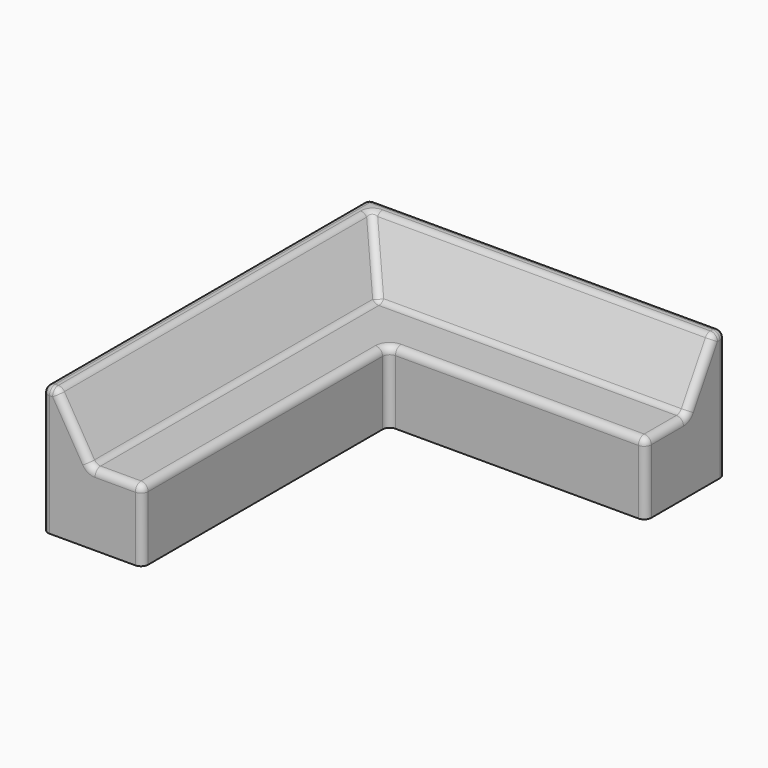
from build123d import *

# Parameters (mm, degrees)
F0_W         = 18
F0_H         = 7
F1_DEPTH     = 5
F2_W         = 21
F2_H         = 4
F3_DEPTH     = 4
F4_T4_DEPTH  = 37.431305486
F4_T9_DEPTH  = 33.931305486
F4_T15_DEPTH = 33.931305486
F4_T21_DEPTH = 37.431305486
F5_R         = 0.5
F6_T1_DEPTH  = 2.8169048105
F6_T3_DEPTH  = 2.8169048105
F6_T5_DEPTH  = 0.2169048105
F6_T7_DEPTH  = 4.0985711369
F6_T9_DEPTH  = 0.2169048105
F6_T11_DEPTH = 4.0985711369
F6_S15_W     = 0.5
F6_S15_H     = 0.5
F6_T16_DEPTH = 0.5
F6_S21_W     = 0.5
F6_S21_H     = 0.5
F6_T22_DEPTH = 0.5
F6_S27_W     = 0.5
F6_S27_H     = 0.5
F6_T28_DEPTH = 0.5
F6_S33_W     = 0.5
F6_S33_H     = 0.5
F6_T34_DEPTH = 0.5
F6_T38_ANGLE = 59.0362434679
F6_T40_ANGLE = 59.0362434679
F6_T42_ANGLE = 59.0362434679
F6_T44_ANGLE = 59.0362434679


# Not quite as in the source:
# - a fillet or chamfer that OpenCascade refuses, or shapes differently, is made with other operations: its cross-section is extruded or revolved along the edge and cut away or added


with BuildPart() as f1:
    # F0 (on Top) → F1 (new body)
    with BuildSketch(Plane.XY):
        Polygon((-41.0881050097, 20.8523701802), (-48.0881050097, 20.8523701802), (-48.0881050097, -7.6476298198), (-41.0881050097, -7.6476298198), (-41.0881050097, 13.8523701802), align=None)
        with Locations((-32.0881050097, 17.3523701802)):
            Rectangle(F0_W, F0_H)
    extrude(amount=F1_DEPTH)

    # F2 (on face) → F3 (join)
    with BuildSketch(Plane.XY.offset(5)):
        Polygon((-44.0881050097, 20.8523701802), (-48.0881050097, 20.8523701802), (-48.0881050097, -7.6476298198), (-44.0881050097, -7.6476298198), (-44.0881050097, 16.8523701802), align=None)
        with Locations((-33.5881050097, 18.8523701802)):
            Rectangle(F2_W, F2_H)
    extrude(amount=F3_DEPTH)

    # F4: chamfer of 5 x 3 on 2 edges, made by hand


with BuildPart() as f4_tool2:
    # F4_s3 → F4_t4 (new body)
    with BuildSketch(Plane.XZ.offset(20.5789353058)):
        Polygon((-44.0881050097, 4), (-47.0881050097, 9), (-44.0881050097, 9), align=None)
    extrude(amount=-F4_T4_DEPTH)

    split(bisect_by=Plane.XY.offset(5), keep=Keep.TOP)


with BuildPart() as f1_1:
    add(f1.part)

    # F4_t1: cut F4_tool2
    add(f4_tool2.part, mode=Mode.SUBTRACT)


with BuildPart() as f4_tool7:
    # F4_s8 → F4_t9 (new body)
    with BuildSketch(Plane.YZ.offset(-44.0881050097)):
        Polygon((16.8523701802, 4), (19.8523701802, 9), (16.8523701802, 9), align=None)
    extrude(amount=F4_T9_DEPTH)

    split(bisect_by=Plane.XY.offset(5), keep=Keep.TOP)


with BuildPart() as f1_2:
    add(f1_1.part)

    # F4_t6: cut F4_tool7
    add(f4_tool7.part, mode=Mode.SUBTRACT)


with BuildPart() as f4_tool13:
    # F4_s14 → F4_t15 (new body)
    with BuildSketch(Plane.YZ.offset(-57.0194104957)):
        Polygon((16.8523701802, 4), (19.8523701802, 9), (16.8523701802, 9), align=None)
    extrude(amount=F4_T15_DEPTH)

    split(bisect_by=Plane.YZ.offset(-48.0881050097), keep=Keep.TOP)

    split(bisect_by=Plane.YZ.offset(-44.0881050097), keep=Keep.BOTTOM)

    split(bisect_by=Plane.XY.offset(5), keep=Keep.TOP)


with BuildPart() as f4_tool19:
    # F4_s20 → F4_t21 (new body)
    with BuildSketch(Plane.XZ.offset(7.6476298198)):
        Polygon((-44.0881050097, 4), (-47.0881050097, 9), (-44.0881050097, 9), align=None)
    extrude(amount=-F4_T21_DEPTH)

    split(bisect_by=Plane.XZ.offset(-16.8523701802), keep=Keep.BOTTOM)

    split(bisect_by=Plane.XY.offset(5), keep=Keep.TOP)

    split(bisect_by=Plane.XZ.offset(-20.8523701802), keep=Keep.TOP)


with BuildPart() as f4_tool13_1:
    add(f4_tool13.part)

    # F4_t25: intersect F4_tool19
    add(f4_tool19.part, mode=Mode.INTERSECT)


with BuildPart() as f1_3:
    add(f1_2.part)

    # F4_t11: cut F4_tool13
    add(f4_tool13_1.part, mode=Mode.SUBTRACT)

    # F5
    f5_edges = [f1_3.edges().sort_by_distance(p)[0] for p in [
        (-48.088105, -7.64763, 4.5),
        (-41.088105, -7.64763, 2.5),
        (-41.088105, 13.85237, 2.5),
        (-23.088105, 13.85237, 2.5),
        (-23.088105, 20.85237, 4.5),
        (-35.588105, 20.85237, 9),
        (-35.088105, 19.85237, 9),
        (-47.088105, 6.10237, 9),
        (-45.888105, 18.65237, 7),
        (-33.888105, 17.45237, 5),
        (-44.688105, 4.90237, 5),
        (-41.088105, 3.10237, 5),
        (-32.088105, 13.85237, 5),
        (-48.088105, 6.60237, 9),
        (-48.088105, 20.85237, 4.5),
    ]]
    fillet(f5_edges, radius=F5_R)

    # F6: fillet of radius 0.5 on 10 edges, made by hand

    # F6_s2 → F6_t1 (cut)
    with BuildSketch(Plane.YZ.offset(-44.4050098202)):
        with BuildLine():
            ThreePointArc((-7.6476298198, 4.5), (-7.5011832104, 4.8535533906), (-7.1476298198, 5))
            Line((-7.1476298198, 5), (-7.6476298198, 5))
            Line((-7.6476298198, 5), (-7.6476298198, 4.5))
        make_face()
    extrude(amount=F6_T1_DEPTH, mode=Mode.SUBTRACT)

    # F6_s4 → F6_t3 (cut)
    with BuildSketch(Plane.XZ.offset(-17.1692749907)):
        with BuildLine():
            ThreePointArc((-23.0881050097, 4.5), (-23.2345516191, 4.8535533906), (-23.5881050097, 5))
            Line((-23.5881050097, 5), (-23.0881050097, 5))
            Line((-23.0881050097, 5), (-23.0881050097, 4.5))
        make_face()
    extrude(amount=F6_T3_DEPTH, mode=Mode.SUBTRACT)

    # F6_s6 → F6_t5 (cut)
    with BuildSketch(Plane.YZ.offset(-47.5881050097)):
        with BuildLine():
            ThreePointArc((-7.6476298198, 8.5), (-7.5011832104, 8.8535533906), (-7.1476298198, 9))
            Line((-7.1476298198, 9), (-7.6476298198, 9))
            Line((-7.6476298198, 9), (-7.6476298198, 8.5))
        make_face()
    extrude(amount=F6_T5_DEPTH, mode=Mode.SUBTRACT)

    # F6_s8 → F6_t7 (cut)
    with BuildSketch(Plane(origin=(-16.2894353468, 0, 27.1490589114), x_dir=(0, 1, 0), z_dir=(0.5144957554, 0, -0.8574929257))):
        with BuildLine():
            ThreePointArc((-7.6476298198, -36.2472551322), (-7.5011832104, -35.8937017416), (-7.1476298198, -35.7472551322))
            Line((-7.1476298198, -35.7472551322), (-7.6476298198, -35.7472551322))
            Line((-7.6476298198, -35.7472551322), (-7.6476298198, -36.2472551322))
        make_face()
    extrude(amount=F6_T7_DEPTH, mode=Mode.SUBTRACT)

    # F6_s10 → F6_t9 (cut)
    with BuildSketch(Plane.XZ.offset(-20.3523701802)):
        with BuildLine():
            ThreePointArc((-23.0881050097, 8.5), (-23.2345516191, 8.8535533906), (-23.5881050097, 9))
            Line((-23.5881050097, 9), (-23.0881050097, 9))
            Line((-23.0881050097, 9), (-23.0881050097, 8.5))
        make_face()
    extrude(amount=F6_T9_DEPTH, mode=Mode.SUBTRACT)

    # F6_s12 → F6_t11 (cut)
    with BuildSketch(Plane(origin=(0, 6.971278674, 11.61879779), x_dir=(1, 0, 0), z_dir=(0, 0.5144957554, 0.8574929257))):
        with BuildLine():
            ThreePointArc((-23.0881050097, 12.8928051893), (-23.2345516191, 12.5392517987), (-23.5881050097, 12.3928051893))
            Line((-23.5881050097, 12.3928051893), (-23.0881050097, 12.3928051893))
            Line((-23.0881050097, 12.3928051893), (-23.0881050097, 12.8928051893))
        make_face()
    extrude(amount=F6_T11_DEPTH, mode=Mode.SUBTRACT)


with BuildPart() as f6_tool14:
    # F6_s15 → F6_t16 (new body)
    with BuildSketch(Plane.YZ.offset(-23.5881050097)):
        with Locations((20.6023701802, 8.75)):
            Rectangle(F6_S15_W, F6_S15_H)
    extrude(amount=F6_T16_DEPTH)

    # F6_s17 → F6_t18 (revolve, cut)
    with BuildSketch(Plane(origin=(-23.5881050097, 20.3523701802, 8.5), x_dir=(0, -0.7071067812, -0.7071067812), z_dir=(0, -0.7071067812, 0.7071067812))):
        with BuildLine():
            ThreePointArc((0, -0.5), (0.5, 0), (0, 0.5))
            Line((0, 0.5), (0, -0.5))
        make_face()
    revolve(axis=Axis((-23.5881050097, 20.3523701802, 8.5), (1, 0, 0)), mode=Mode.SUBTRACT)


with BuildPart() as f1_4:
    add(f1_3.part)

    # F6_t13: cut F6_tool14
    add(f6_tool14.part, mode=Mode.SUBTRACT)


with BuildPart() as f6_tool20:
    # F6_s21 → F6_t22 (new body)
    with BuildSketch(Plane.XZ.offset(7.1476298198)):
        with Locations((-47.8381050097, 8.75)):
            Rectangle(F6_S21_W, F6_S21_H)
    extrude(amount=F6_T22_DEPTH)

    # F6_s23 → F6_t24 (revolve, cut)
    with BuildSketch(Plane(origin=(-47.5881050097, -7.1476298198, 8.5), x_dir=(0.7071067812, 0, -0.7071067812), z_dir=(-0.7071067812, 0, -0.7071067812))):
        with BuildLine():
            ThreePointArc((0, -0.5), (0.5, 0), (0, 0.5))
            Line((0, 0.5), (0, -0.5))
        make_face()
    revolve(axis=Axis((-47.5881050097, -7.1476298198, 8.5), (0, -1, 0)), mode=Mode.SUBTRACT)


with BuildPart() as f1_5:
    add(f1_4.part)

    # F6_t19: cut F6_tool20
    add(f6_tool20.part, mode=Mode.SUBTRACT)


with BuildPart() as f6_tool26:
    # F6_s27 → F6_t28 (new body)
    with BuildSketch(Plane.YZ.offset(-23.5881050097)):
        with Locations((14.1023701802, 4.75)):
            Rectangle(F6_S27_W, F6_S27_H)
    extrude(amount=F6_T28_DEPTH)

    # F6_s29 → F6_t30 (revolve, cut)
    with BuildSketch(Plane(origin=(-23.5881050097, 14.3523701802, 4.5), x_dir=(0, 0.7071067812, -0.7071067812), z_dir=(0, -0.7071067812, -0.7071067812))):
        with BuildLine():
            ThreePointArc((0, -0.5), (0.5, 0), (0, 0.5))
            Line((0, 0.5), (0, -0.5))
        make_face()
    revolve(axis=Axis((-23.5881050097, 14.3523701802, 4.5), (1, 0, 0)), mode=Mode.SUBTRACT)


with BuildPart() as f1_6:
    add(f1_5.part)

    # F6_t25: cut F6_tool26
    add(f6_tool26.part, mode=Mode.SUBTRACT)


with BuildPart() as f6_tool32:
    # F6_s33 → F6_t34 (new body)
    with BuildSketch(Plane.XZ.offset(7.1476298198)):
        with Locations((-41.3381050097, 4.75)):
            Rectangle(F6_S33_W, F6_S33_H)
    extrude(amount=F6_T34_DEPTH)

    # F6_s35 → F6_t36 (revolve, cut)
    with BuildSketch(Plane(origin=(-41.5881050097, -7.1476298198, 4.5), x_dir=(-0.7071067812, 0, -0.7071067812), z_dir=(-0.7071067812, 0, 0.7071067812))):
        with BuildLine():
            ThreePointArc((0, -0.5), (0.5, 0), (0, 0.5))
            Line((0, 0.5), (0, -0.5))
        make_face()
    revolve(axis=Axis((-41.5881050097, -7.1476298198, 4.5), (0, -1, 0)), mode=Mode.SUBTRACT)


with BuildPart() as f1_7:
    add(f1_6.part)

    # F6_t31: cut F6_tool32
    add(f6_tool32.part, mode=Mode.SUBTRACT)

    # F6_s37 → F6_t38 (revolve, cut)
    with BuildSketch(Plane(origin=(-16.2894353468, 0, 27.1490589114), x_dir=(0, 1, 0), z_dir=(0.5144957554, 0, -0.8574929257))):
        with BuildLine():
            ThreePointArc((-7.6476298198, -36.2472551322), (-7.5011832104, -35.8937017416), (-7.1476298198, -35.7472551322))
            Line((-7.1476298198, -35.7472551322), (-7.6476298198, -35.7472551322))
            Line((-7.6476298198, -35.7472551322), (-7.6476298198, -36.2472551322))
        make_face()
    revolve(axis=Axis((-47.3712001992, -7.6476298198, 8.5), (0, -1, 0)), revolution_arc=F6_T38_ANGLE, mode=Mode.SUBTRACT)

    # F6_s39 → F6_t40 (revolve, cut)
    with BuildSketch(Plane(origin=(-14.1807378936, 0, 23.634563156), x_dir=(0, 1, 0), z_dir=(-0.5144957554, 0, 0.8574929257))):
        with BuildLine():
            ThreePointArc((-7.6476298198, 36.2472551322), (-7.5011832104, 35.8937017416), (-7.1476298198, 35.7472551322))
            Line((-7.1476298198, 35.7472551322), (-7.6476298198, 35.7472551322))
            Line((-7.6476298198, 35.7472551322), (-7.6476298198, 36.2472551322))
        make_face()
    revolve(axis=Axis((-44.4050098202, -7.6476298198, 5.5), (0, -1, 0)), revolution_arc=F6_T40_ANGLE, mode=Mode.SUBTRACT)

    # F6_s41 → F6_t42 (revolve, cut)
    with BuildSketch(Plane(origin=(0, 6.971278674, 11.61879779), x_dir=(1, 0, 0), z_dir=(0, 0.5144957554, 0.8574929257))):
        with BuildLine():
            ThreePointArc((-23.0881050097, 12.8928051893), (-23.2345516191, 12.5392517987), (-23.5881050097, 12.3928051893))
            Line((-23.5881050097, 12.3928051893), (-23.0881050097, 12.3928051893))
            Line((-23.0881050097, 12.3928051893), (-23.0881050097, 12.8928051893))
        make_face()
    revolve(axis=Axis((-23.0881050097, 17.1692749907, 5.5), (-1, 0, 0)), revolution_arc=F6_T42_ANGLE, mode=Mode.SUBTRACT)

    # F6_s43 → F6_t44 (revolve, cut)
    with BuildSketch(Plane(origin=(0, 9.0799761273, 15.1332935454), x_dir=(1, 0, 0), z_dir=(0, -0.5144957554, -0.8574929257))):
        with BuildLine():
            ThreePointArc((-23.0881050097, -12.8928051893), (-23.2345516191, -12.5392517987), (-23.5881050097, -12.3928051893))
            Line((-23.5881050097, -12.3928051893), (-23.0881050097, -12.3928051893))
            Line((-23.0881050097, -12.3928051893), (-23.0881050097, -12.8928051893))
        make_face()
    revolve(axis=Axis((-23.0881050097, 20.1354653697, 8.5), (-1, 0, 0)), revolution_arc=F6_T44_ANGLE, mode=Mode.SUBTRACT)


solid = f1_7.part
